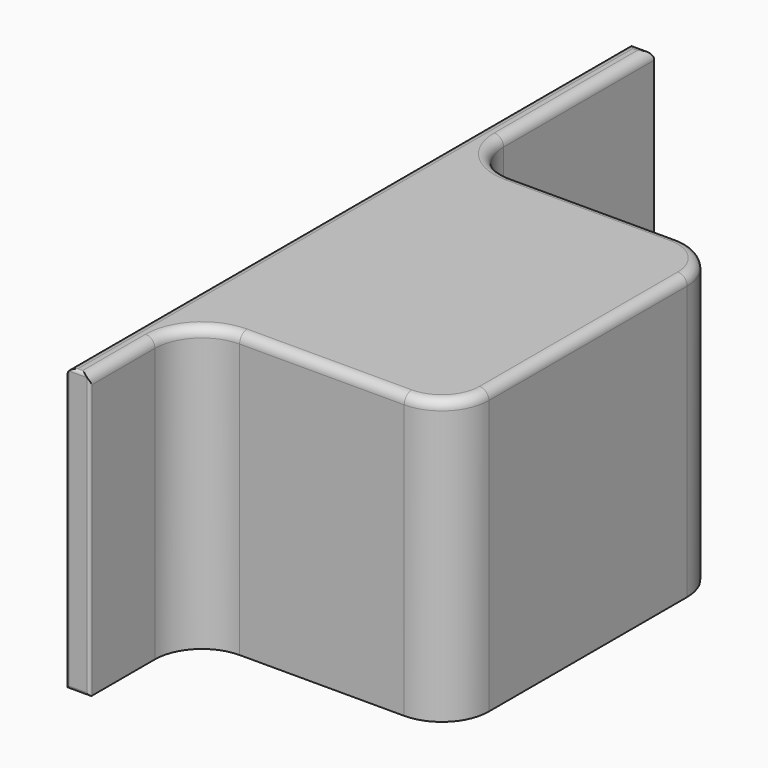
from build123d import *

# Parameters (mm, degrees)
F1_DEPTH     = 152.908
F2_R         = 25.4
F3_R         = 1.5875
F4_T1_DEPTH  = 55.1097300731
F4_T3_DEPTH  = 404.8125
F4_T5_DEPTH  = 88.9
F4_T7_DEPTH  = 38.1
F4_T9_DEPTH  = 114.3
F4_T11_DEPTH = 133.8027699269
F4_T14_ANGLE = 90
F4_T16_ANGLE = 90
F4_T18_ANGLE = 90
F4_T20_ANGLE = 90


# Not quite as in the source:
# - a fillet or chamfer that OpenCascade refuses, or shapes differently, is made with other operations: its cross-section is extruded or revolved along the edge and cut away or added


with BuildPart() as f1:
    # F0 (on Top) → F1 (new body)
    with BuildSketch(Plane.XY):
        Polygon((-148.8164286077, -93.2749655156), (-136.1164286077, -93.2749655156), (-136.1164286077, -23.8777354426), (3.5835713923, -23.8777354426), (3.5835713923, 160.7250344844), (-136.1164286077, 160.7250344844), (-136.1164286077, 287.7250344844), (-148.8164286077, 287.7250344844), align=None)
    extrude(amount=F1_DEPTH)

    # F2
    f2_edges = [f1.edges().sort_by_distance(p)[0] for p in [
        (-136.116429, -23.877735, 76.454),
        (3.583571, -23.877735, 76.454),
        (3.583571, 160.725034, 76.454),
        (-136.116429, 160.725034, 76.454),
    ]]
    fillet(f2_edges, radius=F2_R)

    # F3
    f3_edges = [f1.edges().sort_by_distance(p)[0] for p in [
        (-148.816429, -93.274966, 76.454),
        (-136.116429, -93.274966, 76.454),
        (-142.466429, -93.274966, 0),
        (-142.466429, -93.274966, 152.908),
    ]]
    fillet(f3_edges, radius=F3_R)

    # F4: fillet of radius 5.08 on 12 edges, made by hand

    # F4_s2 → F4_t1 (cut)
    with BuildSketch(Plane.XZ.offset(49.2777354426)):
        with BuildLine():
            ThreePointArc((-136.1164286077, 147.828), (-137.6043261593, 151.4201024484), (-141.1964286077, 152.908))
            Line((-141.1964286077, 152.908), (-136.1164286077, 152.908))
            Line((-136.1164286077, 152.908), (-136.1164286077, 147.828))
        make_face()
    extrude(amount=F4_T1_DEPTH, mode=Mode.SUBTRACT)

    # F4_s4 → F4_t3 (cut)
    with BuildSketch(Plane.XZ.offset(-300.4250344844)):
        with BuildLine():
            ThreePointArc((-143.7364286077, 152.908), (-147.3285310561, 151.4201024484), (-148.8164286077, 147.828))
            Line((-148.8164286077, 147.828), (-148.8164286077, 152.908))
            Line((-148.8164286077, 152.908), (-143.7364286077, 152.908))
        make_face()
    extrude(amount=F4_T3_DEPTH, mode=Mode.SUBTRACT)

    # F4_s6 → F4_t5 (cut)
    with BuildSketch(Plane.YZ.offset(-110.7164286077)):
        with BuildLine():
            ThreePointArc((-18.7977354426, 152.908), (-22.389837891, 151.4201024484), (-23.8777354426, 147.828))
            Line((-23.8777354426, 147.828), (-23.8777354426, 152.908))
            Line((-23.8777354426, 152.908), (-18.7977354426, 152.908))
        make_face()
        with BuildLine():
            ThreePointArc((155.6450344844, 152.908), (159.2371369328, 151.4201024484), (160.7250344844, 147.828))
            Line((160.7250344844, 147.828), (160.7250344844, 152.908))
            Line((160.7250344844, 152.908), (155.6450344844, 152.908))
        make_face()
    extrude(amount=F4_T5_DEPTH, mode=Mode.SUBTRACT)

    # F4_s8 → F4_t7 (cut)
    with BuildSketch(Plane.YZ.offset(-161.5164286077)):
        with BuildLine():
            ThreePointArc((282.6450344844, 152.908), (286.2371369328, 151.4201024484), (287.7250344844, 147.828))
            Line((287.7250344844, 147.828), (287.7250344844, 152.908))
            Line((287.7250344844, 152.908), (282.6450344844, 152.908))
        make_face()
    extrude(amount=F4_T7_DEPTH, mode=Mode.SUBTRACT)

    # F4_s10 → F4_t9 (cut)
    with BuildSketch(Plane.XZ.offset(-300.4250344844)):
        with BuildLine():
            ThreePointArc((-141.1964286077, 152.908), (-137.6043261593, 151.4201024484), (-136.1164286077, 147.828))
            Line((-136.1164286077, 147.828), (-136.1164286077, 152.908))
            Line((-136.1164286077, 152.908), (-141.1964286077, 152.908))
        make_face()
    extrude(amount=F4_T9_DEPTH, mode=Mode.SUBTRACT)

    # F4_s12 → F4_t11 (cut)
    with BuildSketch(Plane.XZ.offset(-135.3250344844)):
        with BuildLine():
            ThreePointArc((-1.4964286077, 152.908), (2.0956738407, 151.4201024484), (3.5835713923, 147.828))
            Line((3.5835713923, 147.828), (3.5835713923, 152.908))
            Line((3.5835713923, 152.908), (-1.4964286077, 152.908))
        make_face()
    extrude(amount=F4_T11_DEPTH, mode=Mode.SUBTRACT)

    # F4_s13 → F4_t14 (revolve, cut)
    with BuildSketch(Plane.XZ.offset(49.2777354426)):
        with BuildLine():
            ThreePointArc((-136.1164286077, 147.828), (-137.6043261593, 151.4201024484), (-141.1964286077, 152.908))
            Line((-141.1964286077, 152.908), (-136.1164286077, 152.908))
            Line((-136.1164286077, 152.908), (-136.1164286077, 147.828))
        make_face()
    revolve(axis=Axis((-110.7164286077, -49.2777354426, 152.908), (0, 0, -1)), revolution_arc=F4_T14_ANGLE, mode=Mode.SUBTRACT)

    # F4_s15 → F4_t16 (revolve, cut)
    with BuildSketch(Plane.YZ.offset(-21.8164286077)):
        with BuildLine():
            ThreePointArc((-18.7977354426, 152.908), (-22.389837891, 151.4201024484), (-23.8777354426, 147.828))
            Line((-23.8777354426, 147.828), (-23.8777354426, 152.908))
            Line((-23.8777354426, 152.908), (-18.7977354426, 152.908))
        make_face()
    revolve(axis=Axis((-21.8164286077, 1.5222645574, 152.908), (0, 0, 1)), revolution_arc=F4_T16_ANGLE, mode=Mode.SUBTRACT)

    # F4_s17 → F4_t18 (revolve, cut)
    with BuildSketch(Plane.YZ.offset(-110.7164286077)):
        with BuildLine():
            ThreePointArc((155.6450344844, 152.908), (159.2371369328, 151.4201024484), (160.7250344844, 147.828))
            Line((160.7250344844, 147.828), (160.7250344844, 152.908))
            Line((160.7250344844, 152.908), (155.6450344844, 152.908))
        make_face()
    revolve(axis=Axis((-110.7164286077, 186.1250344844, 152.908), (0, 0, -1)), revolution_arc=F4_T18_ANGLE, mode=Mode.SUBTRACT)

    # F4_s19 → F4_t20 (revolve, cut)
    with BuildSketch(Plane.XZ.offset(-135.3250344844)):
        with BuildLine():
            ThreePointArc((-1.4964286077, 152.908), (2.0956738407, 151.4201024484), (3.5835713923, 147.828))
            Line((3.5835713923, 147.828), (3.5835713923, 152.908))
            Line((3.5835713923, 152.908), (-1.4964286077, 152.908))
        make_face()
    revolve(axis=Axis((-21.8164286077, 135.3250344844, 152.908), (0, 0, 1)), revolution_arc=F4_T20_ANGLE, mode=Mode.SUBTRACT)


solid = f1.part
